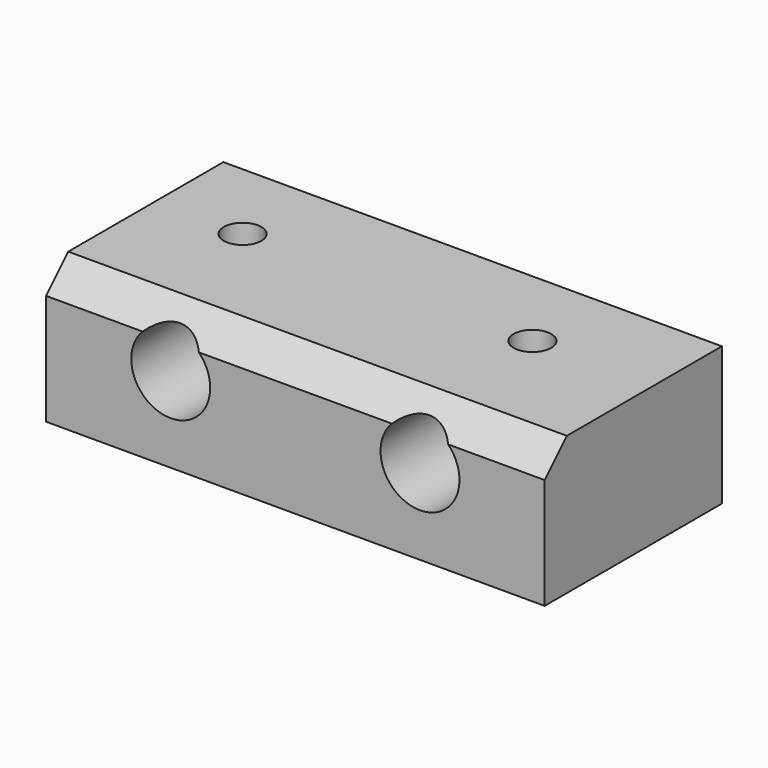
from build123d import *

# Parameters (mm, degrees)
F0_W           = 90
F0_H           = 25
F1_DEPTH       = 40
F3_D           = 8.8
F3_CBORE_D     = 14.25
F3_CBORE_DEPTH = 20
F4_T1_DEPTH    = 115.7168298797
F6_D           = 6.8


# Not quite as in the source:
# - a fillet or chamfer that OpenCascade refuses, or shapes differently, is made with other operations: its cross-section is extruded or revolved along the edge and cut away or added


with BuildPart() as f1:
    # F0 (on Front) → F1 (new body)
    with BuildSketch(Plane.XZ):
        with Locations((45, 12.5)):
            Rectangle(F0_W, F0_H)
    extrude(amount=F1_DEPTH)

    # F3 (through all)
    with Locations(Plane.XZ.offset(40)):
        with Locations((22.5, 15), (67.5, 15)):
            CounterBoreHole(F3_D / 2, F3_CBORE_D / 2, F3_CBORE_DEPTH)

    # F4: chamfer of 5 on 1 edges, made by hand

    # F4_s2 → F4_t1 (cut)
    with BuildSketch(Plane.YZ.offset(-12.8584149398)):
        Polygon((-35, 25), (-40, 20), (-40, 25), align=None)
    extrude(amount=F4_T1_DEPTH, mode=Mode.SUBTRACT)

    # F6 (through all)
    with Locations(Plane.XY.offset(25)):
        with Locations((15.8117040992, -15.4151152819), (68.1231990457, -15.4151152819)):
            Hole(F6_D / 2)


solid = f1.part
